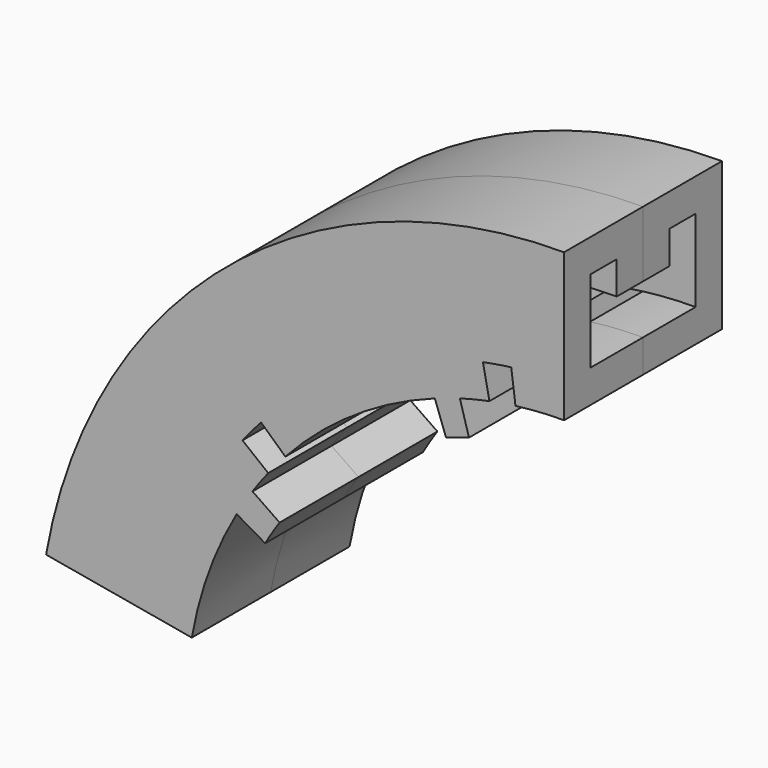
from build123d import *

# Parameters (mm, degrees)
F1_DEPTH = 10
F3_DEPTH = 5
F5_DEPTH = 15
F8_DEPTH = 15
F9_DEPTH = 25


# Not quite as in the source:
# - a feature names something its author has since deleted; it is built from what else it names


with BuildPart() as f1:
    # F0 (on Front) → F1 (new body, symmetric)
    with BuildSketch(Plane.XZ):
        with BuildLine():
            Line((-62.5, -30), (-62.5, 0))
            Line((-62.5, 0), (-75, 0))
            ThreePointArc((-75, 0), (-73.4179734698, -15.3232232767), (-68.7386354243, -30))
            Line((-68.7386354243, -30), (-62.5, -30))
        make_face()
        with BuildLine():
            ThreePointArc((-68.7386354243, -30), (-73.4179734698, -15.3232232767), (-75, 0))
            Line((-75, 0), (-75, -30))
            Line((-75, -30), (-68.7386354243, -30))
        make_face()
        with BuildLine():
            Line((-75, 0), (-62.5, 0))
            ThreePointArc((-62.5, 0), (-44.1941738242, 44.1941738242), (0, 62.5))
            Line((0, 62.5), (0, 75))
            ThreePointArc((0, 75), (-53.033008589, 53.033008589), (-75, 0))
        make_face()
        with BuildLine():
            ThreePointArc((0, 62.5), (23.9177145228, 57.742470782), (44.1941738242, 44.1941738242))
            Line((44.1941738242, 44.1941738242), (44.1941738242, 56.6941738242))
            Line((44.1941738242, 56.6941738242), (49.0995993303, 56.6941738242))
            ThreePointArc((49.0995993303, 56.6941738242), (26.2005435362, 70.274686185), (0, 75))
            Line((0, 75), (0, 62.5))
        make_face()
        with BuildLine():
            Line((44.1941738242, 56.6941738242), (44.1941738242, 44.1941738242))
            Line((44.1941738242, 44.1941738242), (53.033008589, 53.033008589))
            ThreePointArc((53.033008589, 53.033008589), (51.0991040315, 54.8988302897), (49.0995993303, 56.6941738242))
            Line((49.0995993303, 56.6941738242), (44.1941738242, 56.6941738242))
        make_face()
        with BuildLine():
            ThreePointArc((49.0995993303, 56.6941738242), (51.0991040315, 54.8988302897), (53.033008589, 53.033008589))
            ThreePointArc((53.033008589, 53.033008589), (56.9861303035, 48.7604445533), (60.5959982177, 44.1941738242))
            Line((60.5959982177, 44.1941738242), (79.1941738242, 44.1941738242))
            Line((79.1941738242, 44.1941738242), (79.1941738242, 56.6941738242))
            Line((79.1941738242, 56.6941738242), (49.0995993303, 56.6941738242))
        make_face()
        with BuildLine():
            Line((53.033008589, 53.033008589), (44.1941738242, 44.1941738242))
            Line((44.1941738242, 44.1941738242), (60.5959982177, 44.1941738242))
            ThreePointArc((60.5959982177, 44.1941738242), (56.9861303035, 48.7604445533), (53.033008589, 53.033008589))
        make_face()
    extrude(amount=F1_DEPTH, both=True)

    # F2 (on Front) → F3 (cut, symmetric)
    with BuildSketch(Plane.XZ):
        with BuildLine():
            Line((45.9241320293, 52.8296706156), (49.2044271743, 56.6032185167))
            ThreePointArc((49.2044271743, 56.6032185167), (-31.1019931992, 68.2470953157), (-75, 0))
            Line((-75, 0), (-70, 0))
            ThreePointArc((-70, 0), (-29.0285269859, 63.6972889614), (45.9241320293, 52.8296706156))
        make_face()
    extrude(amount=F3_DEPTH, both=True, mode=Mode.SUBTRACT)


with BuildPart() as f5:
    # F4 (on Front) → F5 (new body)
    with BuildSketch(Plane.XZ):
        with BuildLine():
            ThreePointArc((-56.6264457982, 9.9847702158), (-36.960287557, 44.0475554793), (0, 57.5))
            Line((0, 57.5), (0, 80))
            ThreePointArc((0, 80), (-51.4230087749, 61.2835554495), (-78.784620241, 13.8918542134))
            Line((-78.784620241, 13.8918542134), (-56.6264457982, 9.9847702158))
        make_face()
    extrude(amount=F5_DEPTH)

    # F6: cut F1
    add(f1.part, mode=Mode.SUBTRACT)

    # F7 (on face) → F8 (join, through all)
    with BuildSketch(Plane.XZ.offset(15)):
        with BuildLine():
            ThreePointArc((-47.389204942, 32.5655224887), (-48.6302678935, 30.6813794443), (-49.7964607176, 28.75))
            Line((-49.7964607176, 28.75), (-45.4663336987, 26.25))
            ThreePointArc((-45.4663336987, 26.25), (-44.4015489462, 28.0134334057), (-43.2684045123, 29.7337379245))
            Line((-43.2684045123, 29.7337379245), (-47.389204942, 32.5655224887))
        make_face()
        with BuildLine():
            Line((-14.4709611804, 50.4662390368), (-15.8491479595, 55.2725475165))
            ThreePointArc((-15.8491479595, 55.2725475165), (-17.7684771766, 54.685749687), (-19.6661582412, 54.0323256952))
            Line((-19.6661582412, 54.0323256952), (-17.9560575246, 49.3338625913))
            ThreePointArc((-17.9560575246, 49.3338625913), (-16.2233922047, 49.9304671055), (-14.4709611804, 50.4662390368))
        make_face()
    extrude(amount=-F8_DEPTH)

    # F7 (on face) → F9 (cut)
    with BuildSketch(Plane.XZ.offset(15)):
        with BuildLine():
            Line((-48.9153382675, 38.9042373293), (-45.0021112061, 35.7918983429))
            ThreePointArc((-45.0021112061, 35.7918983429), (-43.7255778977, 37.3406459172), (-42.395771708, 38.8438996663))
            Line((-42.395771708, 38.8438996663), (-46.0823605522, 42.221630072))
            ThreePointArc((-46.0823605522, 42.221630072), (-47.5278020627, 40.5876586056), (-48.9153382675, 38.9042373293))
        make_face()
        with BuildLine():
            ThreePointArc((-11.3558821654, 56.3674901006), (-9.3817674339, 56.7294671209), (-7.396222464, 57.0223280239))
            Line((-7.396222464, 57.0223280239), (-8.0393722435, 61.9807913303))
            ThreePointArc((-8.0393722435, 61.9807913303), (-10.1975732978, 61.6624642618), (-12.3433501798, 61.269010979))
            Line((-12.3433501798, 61.269010979), (-11.3558821654, 56.3674901006))
        make_face()
    extrude(amount=-F9_DEPTH, mode=Mode.SUBTRACT)


with BuildPart() as f10_1:
    # F10: instance of F5
    add(f5.part.mirror(Plane.XZ))


solid = Compound([f5.part, f10_1.part])
